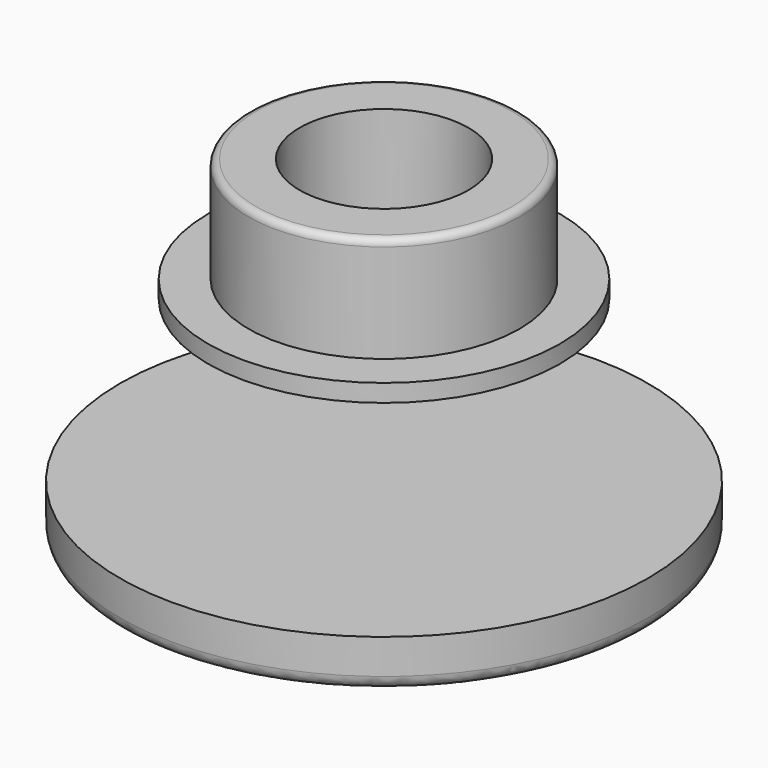
from build123d import *

# Parameters (mm, degrees)
F0_R     = 4.8895
F0_R_2   = 3.048
F1_DEPTH = 3.81
F2_R     = 6.35
F2_R_2   = 4.8895
F2_R_3   = 3.048
F3_DEPTH = 0.635
F6_R     = 0.508
F7_R     = 0.254


with BuildPart() as f1:
    # F0 (on Top) → F1 (new body)
    with BuildSketch(Plane.XY):
        Circle(F0_R)
        Circle(F0_R_2, mode=Mode.SUBTRACT)
    extrude(amount=F1_DEPTH)

    # F2 (on face) → F3 (join)
    with BuildSketch(Plane(origin=(0, 0, 0), x_dir=(1, 0, 0), z_dir=(0, 0, -1))):
        Circle(F2_R)
        Circle(F2_R_2, mode=Mode.SUBTRACT)
        Circle(F2_R_2)
        Circle(F2_R_3, mode=Mode.SUBTRACT)
        Circle(F2_R_3)
    extrude(amount=F3_DEPTH)

    # F7
    f7_edges = [f1.edges().sort_by_distance(p)[0] for p in [
        (-4.8895, 0, 3.81),
    ]]
    fillet(f7_edges, radius=F7_R)


with BuildPart() as f5:
    # F4 (on Front) → F5 (revolve)
    with BuildSketch(Plane.XZ):
        with BuildLine():
            Line((9.525, -6.4157823257), (0, -6.4157823257))
            Line((0, -6.4157823257), (0, -7.0507823257))
            ThreePointArc((0, -7.0507823257), (4.8000755161, -7.403965955), (9.525, -8.3207823257))
            Line((9.525, -8.3207823257), (9.525, -6.4157823257))
        make_face()
    revolve(axis=Axis((0, 0, -0.635), (0, 0, -1)))

    # F6
    f6_edges = [f5.edges().sort_by_distance(p)[0] for p in [
        (-9.525, 0, -8.320782),
    ]]
    fillet(f6_edges, radius=F6_R)


solid = Compound([f1.part, f5.part])
